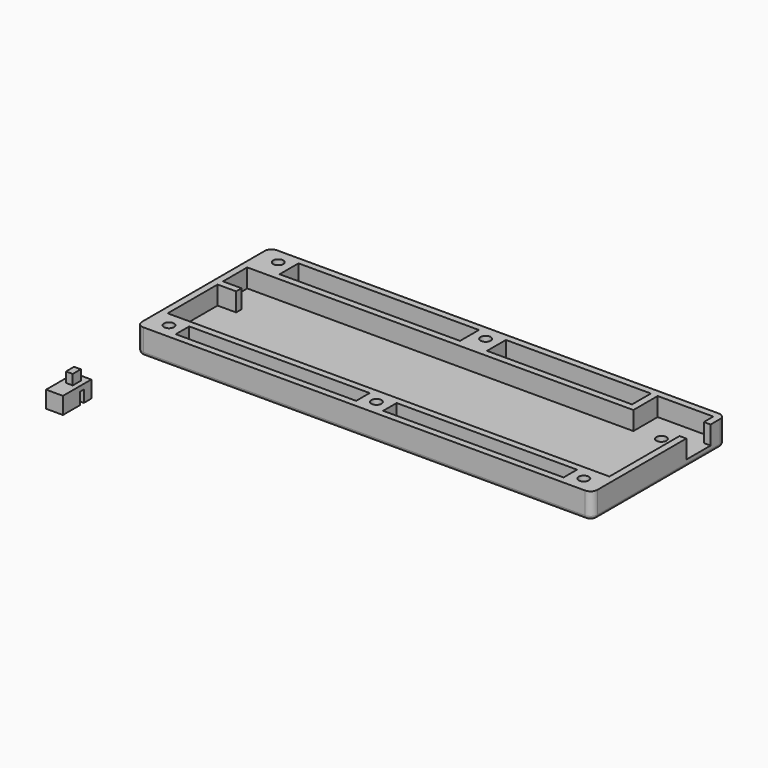
from build123d import *

# Parameters (mm, degrees)
F0_W         = 52
F0_H         = 22
F0_R         = 1.5
F0_W_2       = 5.5
F0_H_2       = 9
F0_H_3       = 18.5
F0_W_3       = 2
F0_W_4       = 48
F0_H_4       = 18
F1_DEPTH     = 2
F0_W_5       = 53.5
F0_H_5       = 7
F0_W_6       = 43
F0_H_6       = 5
F0_H_7       = 2
F0_W_7       = 8
F0_W_8       = 10
F2_DEPTH     = 7.5
F3_W         = 2
F3_H         = 1.5
F4_DEPTH     = 5
F5_DEPTH     = 3.5
F6_W         = 2
F6_H         = 3
F7_DEPTH     = 3
F8_R         = 1
F9_T1_DEPTH  = 12.5
F9_T4_ANGLE  = 90
F9_T6_ANGLE  = 90
F9_T8_ANGLE  = 90
F9_T10_ANGLE = 90
F10_DEPTH    = 2
F11_DEPTH    = 1
F12_DEPTH    = 2.5


# Not quite as in the source:
# - a fillet or chamfer that OpenCascade refuses, or shapes differently, is made with other operations: its cross-section is extruded or revolved along the edge and cut away or added


with BuildPart() as f1:
    # F0 (on Top) → F1 (new body)
    with BuildSketch(Plane.XY):
        Polygon((65.5, 15.75), (65.5, 19.25), (49, 19.25), (49, 10.25), (-60, 10.25), (-60, 1.25), (-60, -0.75), (-60, -19.25), (-4, -19.25), (4, -19.25), (57.5, -19.25), (65.5, -19.25), (65.5, 6.75), align=None)
        with Locations((0, -4.25)):
            Rectangle(F0_W, F0_H, mode=Mode.SUBTRACT)
        with Locations((56.5, 11.25)):
            Circle(F0_R, mode=Mode.SUBTRACT)
        with Locations((-62.75, 5.75)):
            Rectangle(F0_W_2, F0_H_2)
        with Locations((-62.75, -10)):
            Rectangle(F0_W_2, F0_H_3)
        with Locations((66.5, 11.25)):
            Rectangle(F0_W_3, F0_H_2)
        with Locations((0, -4.25)):
            Rectangle(F0_W, F0_H)
        with Locations((0, -4.25)):
            Rectangle(F0_W_4, F0_H_4, mode=Mode.SUBTRACT)
    extrude(amount=F1_DEPTH)



with BuildPart() as f1b:
    # F0 (on Top) → F1, piece 2 (new body)
    with BuildSketch(Plane.XY):
        with Locations((-30.75, 15.75)):
            Rectangle(F0_W_5, F0_H_5)
    extrude(amount=F1_DEPTH)


with BuildPart() as f1c:
    # F0 (on Top) → F1, piece 3 (new body)
    with BuildSketch(Plane.XY):
        with Locations((25.5, 15.75)):
            Rectangle(F0_W_6, F0_H_5)
    extrude(amount=F1_DEPTH)


with BuildPart() as f1d:
    # F0 (on Top) → F1, piece 4 (new body)
    with BuildSketch(Plane.XY):
        with Locations((30.75, -23.75)):
            Rectangle(F0_W_5, F0_H_6)
    extrude(amount=F1_DEPTH)


with BuildPart() as f1e:
    # F0 (on Top) → F1, piece 5 (new body)
    with BuildSketch(Plane.XY):
        with Locations((-30.75, -23.75)):
            Rectangle(F0_W_5, F0_H_6)
    extrude(amount=F1_DEPTH)


with BuildPart() as f1_1:
    add(f1.part)

    add(f1b.part)  # F2 merges F1b

    add(f1c.part)  # F2 merges F1c

    add(f1d.part)  # F2 merges F1d

    add(f1e.part)  # F2 merges F1e
    # F0 (on Top) → F2 (join)
    with BuildSketch(Plane.XY):
        Polygon((49, 10.25), (49, 19.25), (47, 19.25), (47, 12.25), (4, 12.25), (-4, 12.25), (-57.5, 12.25), (-65.5, 12.25), (-65.5, 10.25), (-60, 10.25), align=None)
        with Locations((-66.5, 11.25)):
            Rectangle(F0_W_3, F0_H_7)
        with Locations((-66.5, 5.75)):
            Rectangle(F0_W_3, F0_H_2)
        with Locations((-66.5, 0.25)):
            Rectangle(F0_W_3, F0_H_7)
        with Locations((-62.75, 0.25)):
            Rectangle(F0_W_2, F0_H_7)
        Polygon((-65.5, -19.25), (-65.5, -0.75), (-67.5, -0.75), (-67.5, -21.25), (-57.5, -21.25), (-4, -21.25), (-4, -19.25), (-60, -19.25), align=None)
        Polygon((49, 19.25), (65.5, 19.25), (65.5, 15.75), (67.5, 15.75), (67.5, 21.25), (47, 21.25), (47, 19.25), align=None)
        with Locations((0, -20.25)):
            Rectangle(F0_W_7, F0_H_7)
        with Locations((0, -23.75)):
            Rectangle(F0_W_7, F0_H_6)
        with Locations((0, -23.75)):
            Circle(F0_R, mode=Mode.SUBTRACT)
        with Locations((30.75, -20.25)):
            Rectangle(F0_W_5, F0_H_7)
        with Locations((0, -27.25)):
            Rectangle(F0_W_7, F0_H_7)
        with Locations((-30.75, -27.25)):
            Rectangle(F0_W_5, F0_H_7)
        with Locations((30.75, -27.25)):
            Rectangle(F0_W_5, F0_H_7)
        with Locations((-62.5, -23.75)):
            Rectangle(F0_W_8, F0_H_6)
        with Locations((-61.5, -23.75)):
            Circle(F0_R, mode=Mode.SUBTRACT)
        with Locations((-62.5, -27.25)):
            Rectangle(F0_W_8, F0_H_7)
        Polygon((67.5, 6.75), (65.5, 6.75), (65.5, -19.25), (57.5, -19.25), (57.5, -21.25), (67.5, -21.25), align=None)
        with Locations((62.5, -23.75)):
            Rectangle(F0_W_8, F0_H_6)
        with Locations((61.5, -23.75)):
            Circle(F0_R, mode=Mode.SUBTRACT)
        with Locations((62.5, -27.25)):
            Rectangle(F0_W_8, F0_H_7)
        with Locations((25.5, 20.25)):
            Rectangle(F0_W_6, F0_H_7)
        with Locations((0, 20.25)):
            Rectangle(F0_W_7, F0_H_7)
        with Locations((0, 15.75)):
            Rectangle(F0_W_7, F0_H_5)
        with Locations((0, 16.75)):
            Circle(F0_R, mode=Mode.SUBTRACT)
        with Locations((-61.5, 15.75)):
            Rectangle(F0_W_7, F0_H_5)
        with Locations((-61.5, 16.75)):
            Circle(F0_R, mode=Mode.SUBTRACT)
        Polygon((-65.5, 19.25), (-57.5, 19.25), (-57.5, 21.25), (-67.5, 21.25), (-67.5, 12.25), (-65.5, 12.25), align=None)
        with Locations((-30.75, 20.25)):
            Rectangle(F0_W_5, F0_H_7)
    extrude(amount=F2_DEPTH)

    # F8
    f8_edges = [f1_1.edges().sort_by_distance(p)[0] for p in [
        (67.5, -3.5, 0),
        (0, -28.25, 0),
        (0, 21.25, 0),
        (-67.5, -3.5, 0),
    ]]
    fillet(f8_edges, radius=F8_R)

    # F9: fillet of radius 2 on 4 edges, made by hand

    # F9_s2 → F9_t1 (cut)
    with BuildSketch(Plane.XY):
        with BuildLine():
            ThreePointArc((67.5, -26.25), (66.9142135624, -27.6642135624), (65.5, -28.25))
            Line((65.5, -28.25), (67.5, -28.25))
            Line((67.5, -28.25), (67.5, -26.25))
        make_face()
        with BuildLine():
            ThreePointArc((67.5, 19.25), (66.9142135624, 20.6642135624), (65.5, 21.25))
            Line((65.5, 21.25), (67.5, 21.25))
            Line((67.5, 21.25), (67.5, 19.25))
        make_face()
        with BuildLine():
            ThreePointArc((-65.5, 21.25), (-66.9142135624, 20.6642135624), (-67.5, 19.25))
            Line((-67.5, 19.25), (-67.5, 21.25))
            Line((-67.5, 21.25), (-65.5, 21.25))
        make_face()
        with BuildLine():
            ThreePointArc((-65.5, -28.25), (-66.9142135624, -27.6642135624), (-67.5, -26.25))
            Line((-67.5, -26.25), (-67.5, -28.25))
            Line((-67.5, -28.25), (-65.5, -28.25))
        make_face()
    extrude(amount=F9_T1_DEPTH, mode=Mode.SUBTRACT)

    # F9_s3 → F9_t4 (revolve, cut)
    with BuildSketch(Plane.YZ.offset(-65.5)):
        with BuildLine():
            ThreePointArc((-27.25, 0), (-27.9571067812, 0.2928932188), (-28.25, 1))
            Line((-28.25, 1), (-28.25, 0))
            Line((-28.25, 0), (-27.25, 0))
        make_face()
    revolve(axis=Axis((-65.5, -26.25, 0), (0, 0, -1)), revolution_arc=F9_T4_ANGLE, mode=Mode.SUBTRACT)

    # F9_s5 → F9_t6 (revolve, cut)
    with BuildSketch(Plane.XZ.offset(-19.25)):
        with BuildLine():
            ThreePointArc((-66.5, 0), (-67.2071067812, 0.2928932188), (-67.5, 1))
            Line((-67.5, 1), (-67.5, 0))
            Line((-67.5, 0), (-66.5, 0))
        make_face()
    revolve(axis=Axis((-65.5, 19.25, 0), (0, 0, -1)), revolution_arc=F9_T6_ANGLE, mode=Mode.SUBTRACT)

    # F9_s7 → F9_t8 (revolve, cut)
    with BuildSketch(Plane.YZ.offset(65.5)):
        with BuildLine():
            ThreePointArc((20.25, 0), (20.9571067812, 0.2928932188), (21.25, 1))
            Line((21.25, 1), (21.25, 0))
            Line((21.25, 0), (20.25, 0))
        make_face()
    revolve(axis=Axis((65.5, 19.25, 0), (0, 0, -1)), revolution_arc=F9_T8_ANGLE, mode=Mode.SUBTRACT)

    # F9_s9 → F9_t10 (revolve, cut)
    with BuildSketch(Plane.XZ.offset(26.25)):
        with BuildLine():
            ThreePointArc((66.5, 0), (67.2071067812, 0.2928932188), (67.5, 1))
            Line((67.5, 1), (67.5, 0))
            Line((67.5, 0), (66.5, 0))
        make_face()
    revolve(axis=Axis((65.5, -26.25, 0), (0, 0, -1)), revolution_arc=F9_T10_ANGLE, mode=Mode.SUBTRACT)

    # F0 (on Top) → F10 (join)
    with BuildSketch(Plane.XY):
        with Locations((0, -4.25)):
            Rectangle(F0_W_4, F0_H_4)
    extrude(amount=F10_DEPTH)


with BuildPart() as f4:
    # F3 (on Top) → F4 (new body)
    with BuildSketch(Plane.XY):
        Polygon((-61.5765547214, -49.9684383273), (-66.5765547214, -49.9684383273), (-66.5765547214, -61.9684383273), (-61.5765547214, -61.9684383273), (-61.5765547214, -56.7184383273), (-63.5765547214, -56.7184383273), (-63.5765547214, -55.2184383273), (-61.5765547214, -55.2184383273), align=None)
        with Locations((-62.5765547214, -55.9684383273)):
            Rectangle(F3_W, F3_H)
    extrude(amount=F4_DEPTH)

    # F3 (on Top) → F5 (cut)
    with BuildSketch(Plane.XY):
        with Locations((-62.5765547214, -55.9684383273)):
            Rectangle(F3_W, F3_H)
    extrude(amount=F5_DEPTH, mode=Mode.SUBTRACT)

    # F6 (on face) → F7 (join)
    with BuildSketch(Plane.XY.offset(5)):
        with Locations((-64.0765547214, -55.9684383273)):
            Rectangle(F6_W, F6_H)
    extrude(amount=F7_DEPTH)

    # F11 (add): a face of the model
    f11_faces = [f4.faces().sort_by_distance(p)[0] for p in [
        (-64.0765547214, -61.9684383273, 2.5),
    ]]
    extrude(f11_faces, amount=F11_DEPTH)

    # F12 (cut): a face of the model
    f12_faces = [f4.faces().sort_by_distance(p)[0] for p in [
        (-64.0765547214, -49.9684383273, 2.5),
    ]]
    extrude(f12_faces, amount=-F12_DEPTH, mode=Mode.SUBTRACT)


solid = Compound([f1_1.part, f4.part])
